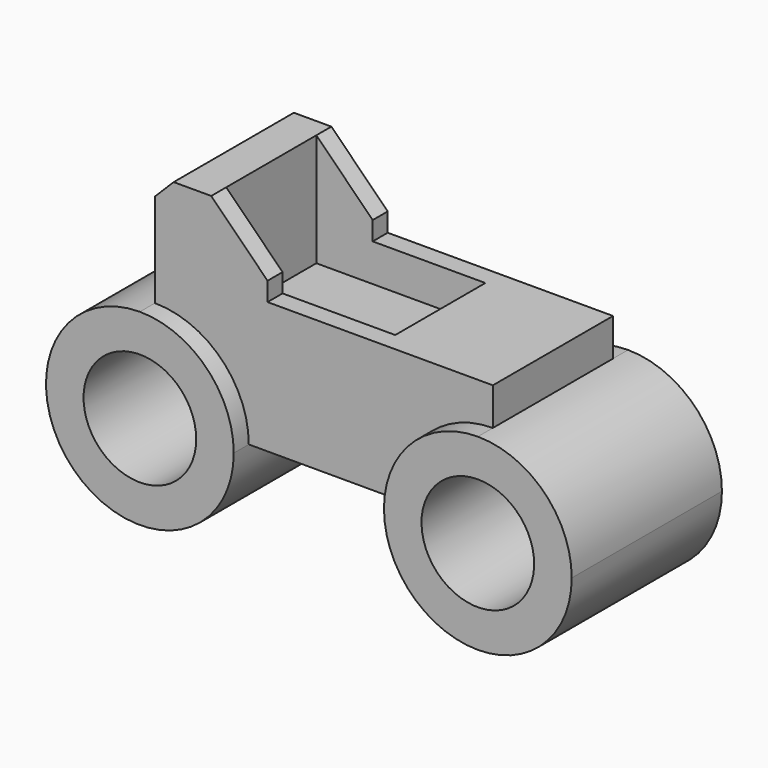
from build123d import *
from build123d import SkipClean  # not in build123d's __all__

# Parameters (mm, degrees)
F1_DEPTH = 50
F2_DEPTH = 5
F4_DEPTH = 5
F5_W     = 30
F5_H     = 30
F6_DEPTH = 10
F7_W     = 30
F7_H     = 20.1446080953
F8_DEPTH = 15


with BuildPart() as f1:
    # F0 (on Front) → F1 (new body)
    with BuildSketch(Plane.XZ):
        with BuildLine():
            Line((-34.2131151259, 22.4876786768), (-44.2131151259, 22.4876786768))
            Line((-44.2131151259, 22.4876786768), (-49.2131151259, 17.4876786768))
            Line((-49.2131151259, 17.4876786768), (-49.2131151259, -7.5123213232))
            ThreePointArc((-49.2131151259, -7.5123213232), (-31.5354455962, -14.8346517935), (-24.2131151259, -32.5123213232))
            Line((-24.2131151259, -32.5123213232), (15.7868848741, -32.5123213232))
            ThreePointArc((15.7868848741, -32.5123213232), (23.1092153444, -14.8346517935), (40.7868848741, -7.5123213232))
            Line((40.7868848741, -7.5123213232), (40.7868848741, 2.4876786768))
            Line((40.7868848741, 2.4876786768), (-19.2131151259, 2.4876786768))
            Line((-19.2131151259, 2.4876786768), (-19.2131151259, 7.4876786768))
            Line((-19.2131151259, 7.4876786768), (-34.2131151259, 22.4876786768))
        make_face()
        with BuildLine():
            Line((-49.2131151259, -17.5123213232), (-49.2131151259, -7.5123213232))
            ThreePointArc((-49.2131151259, -7.5123213232), (-66.8907846556, -50.1899908528), (-24.2131151259, -32.5123213232))
            Line((-24.2131151259, -32.5123213232), (-34.2131151259, -32.5123213232))
            ThreePointArc((-34.2131151259, -32.5123213232), (-59.8197168437, -43.118923041), (-49.2131151259, -17.5123213232))
        make_face()
        with BuildLine():
            ThreePointArc((-24.2131151259, -32.5123213232), (-31.5354455962, -14.8346517935), (-49.2131151259, -7.5123213232))
            Line((-49.2131151259, -7.5123213232), (-49.2131151259, -17.5123213232))
            ThreePointArc((-49.2131151259, -17.5123213232), (-38.6065134081, -21.9057196054), (-34.2131151259, -32.5123213232))
            Line((-34.2131151259, -32.5123213232), (-24.2131151259, -32.5123213232))
        make_face()
        with BuildLine():
            ThreePointArc((40.7868848741, -7.5123213232), (23.1092153444, -14.8346517935), (15.7868848741, -32.5123213232))
            Line((15.7868848741, -32.5123213232), (25.7868848741, -32.5123213232))
            ThreePointArc((25.7868848741, -32.5123213232), (30.1802831563, -21.9057196054), (40.7868848741, -17.5123213232))
            Line((40.7868848741, -17.5123213232), (40.7868848741, -7.5123213232))
        make_face()
        with BuildLine():
            Line((25.7868848741, -32.5123213232), (15.7868848741, -32.5123213232))
            ThreePointArc((15.7868848741, -32.5123213232), (40.7868848741, -57.5123213232), (65.7868848741, -32.5123213232))
            ThreePointArc((65.7868848741, -32.5123213232), (58.4645544038, -14.8346517935), (40.7868848741, -7.5123213232))
            Line((40.7868848741, -7.5123213232), (40.7868848741, -17.5123213232))
            ThreePointArc((40.7868848741, -17.5123213232), (51.3934865919, -21.9057196054), (55.7868848741, -32.5123213232))
            ThreePointArc((55.7868848741, -32.5123213232), (40.7868848741, -47.5123213232), (25.7868848741, -32.5123213232))
        make_face()
    extrude(amount=F1_DEPTH)

    # F0 (on Front) → F2 (cut)
    with BuildSketch(Plane.XZ):
        with BuildLine():
            Line((-34.2131151259, 22.4876786768), (-44.2131151259, 22.4876786768))
            Line((-44.2131151259, 22.4876786768), (-49.2131151259, 17.4876786768))
            Line((-49.2131151259, 17.4876786768), (-49.2131151259, -7.5123213232))
            ThreePointArc((-49.2131151259, -7.5123213232), (-31.5354455962, -14.8346517935), (-24.2131151259, -32.5123213232))
            Line((-24.2131151259, -32.5123213232), (15.7868848741, -32.5123213232))
            ThreePointArc((15.7868848741, -32.5123213232), (23.1092153444, -14.8346517935), (40.7868848741, -7.5123213232))
            Line((40.7868848741, -7.5123213232), (40.7868848741, 2.4876786768))
            Line((40.7868848741, 2.4876786768), (-19.2131151259, 2.4876786768))
            Line((-19.2131151259, 2.4876786768), (-19.2131151259, 7.4876786768))
            Line((-19.2131151259, 7.4876786768), (-34.2131151259, 22.4876786768))
        make_face()
    extrude(amount=F2_DEPTH, mode=Mode.SUBTRACT)

    # F3 (on face) → F4 (cut)
    with BuildSketch(Plane.XZ.offset(50)):
        with BuildLine():
            Line((-34.2131151259, 22.4876786768), (-44.2131151259, 22.4876786768))
            Line((-44.2131151259, 22.4876786768), (-49.2131151259, 17.4876786768))
            Line((-49.2131151259, 17.4876786768), (-49.2131151259, -7.5123213232))
            ThreePointArc((-49.2131151259, -7.5123213232), (-31.5354455962, -14.8346517935), (-24.2131151259, -32.5123213232))
            Line((-24.2131151259, -32.5123213232), (15.7868848741, -32.5123213232))
            ThreePointArc((15.7868848741, -32.5123213232), (23.1092153444, -14.8346517935), (40.7868848741, -7.5123213232))
            Line((40.7868848741, -7.5123213232), (40.7868848741, 2.4876786768))
            Line((40.7868848741, 2.4876786768), (-19.2131151259, 2.4876786768))
            Line((-19.2131151259, 2.4876786768), (-19.2131151259, 7.4876786768))
            Line((-19.2131151259, 7.4876786768), (-34.2131151259, 22.4876786768))
        make_face()
    with SkipClean():  # cleaning this boolean's faces spoils the solid; the shape is the same uncleaned
        extrude(amount=-F4_DEPTH, mode=Mode.SUBTRACT)

    # F5 (on face) → F6 (cut)
    with BuildSketch(Plane.XY.offset(2.4876786768)):
        with Locations((-4.2131151259, -25)):
            Rectangle(F5_W, F5_H)
    extrude(amount=-F6_DEPTH, mode=Mode.SUBTRACT)

    # F7 (on face) → F8 (cut)
    with BuildSketch(Plane.YZ.offset(-19.2131151259)):
        Polygon((-40, 2.4876786768), (-40, -7.5123213232), (-10, -7.5123213232), (-10, 2.4876786768), (-10, 7.4876786768), (-40, 7.4876786768), align=None)
        with Locations((-25, 17.5599827245)):
            Rectangle(F7_W, F7_H)
    extrude(amount=-F8_DEPTH, mode=Mode.SUBTRACT)


solid = f1.part
